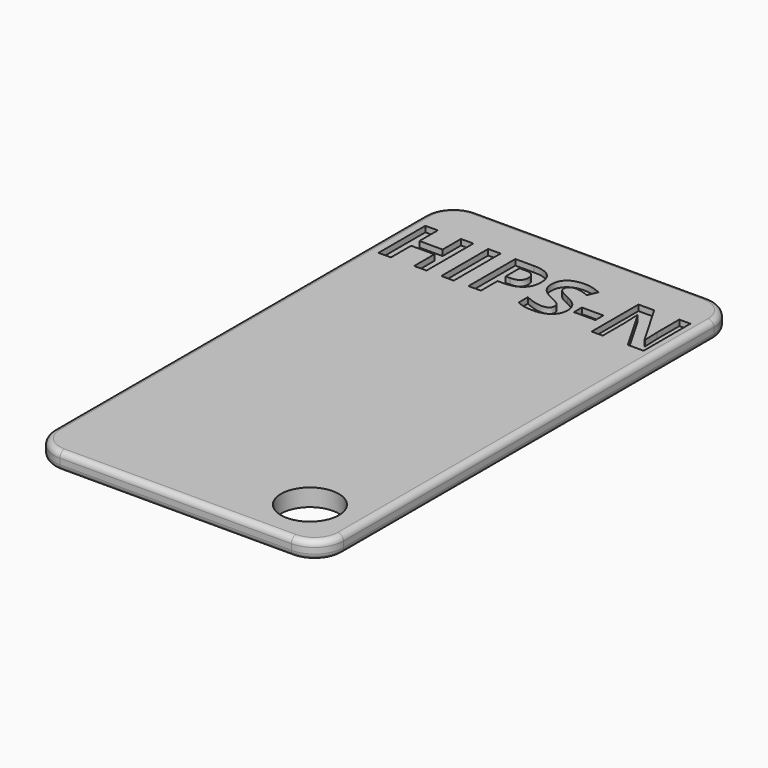
from build123d import *

# Parameters (mm, degrees)
F0_W         = 90
F0_H         = 50
F1_DEPTH     = 3
F2_R         = 1
F3_T1_DEPTH  = 3
F3_T4_ANGLE  = 90
F3_T6_ANGLE  = 90
F3_T8_ANGLE  = 90
F3_T10_ANGLE = 90
F3_T12_ANGLE = 90
F3_T14_ANGLE = 90
F3_T16_ANGLE = 90
F3_T18_ANGLE = 90
F5_ANGLE     = 90
F6_TEXT_SIZE = 14.1815160188
F7_DEPTH     = 1
F8_R         = 5
F9_DEPTH     = 3


# Not quite as in the source:
# - a fillet or chamfer that OpenCascade refuses, or shapes differently, is made with other operations: its cross-section is extruded or revolved along the edge and cut away or added
# - Text() gives the source's letters only with a copy of the font that has no kerning and outlines rounded to 1/6400 em; it was checked with that copy


with BuildPart() as f1:
    # F0 (on Top) → F1 (new body)
    with BuildSketch(Plane.XY):
        Rectangle(F0_W, F0_H)
    extrude(amount=F1_DEPTH)

    # F2
    f2_edges = [f1.edges().sort_by_distance(p)[0] for p in [
        (0, 25, 3),
        (-45, 0, 3),
        (0, -25, 3),
        (45, 0, 3),
        (0, 25, 0),
        (-45, 0, 0),
        (0, -25, 0),
        (45, 0, 0),
    ]]
    fillet(f2_edges, radius=F2_R)

    # F3: fillet of radius 5 on 4 edges, made by hand

    # F3_s2 → F3_t1 (cut)
    with BuildSketch(Plane.XY):
        with BuildLine():
            ThreePointArc((45, -20), (43.5355339059, -23.5355339059), (40, -25))
            Line((40, -25), (45, -25))
            Line((45, -25), (45, -20))
        make_face()
        with BuildLine():
            ThreePointArc((40, 25), (43.5355339059, 23.5355339059), (45, 20))
            Line((45, 20), (45, 25))
            Line((45, 25), (40, 25))
        make_face()
        with BuildLine():
            ThreePointArc((-40, 25), (-43.5355339059, 23.5355339059), (-45, 20))
            Line((-45, 20), (-45, 25))
            Line((-45, 25), (-40, 25))
        make_face()
        with BuildLine():
            ThreePointArc((-45, -20), (-43.5355339059, -23.5355339059), (-40, -25))
            Line((-40, -25), (-45, -25))
            Line((-45, -25), (-45, -20))
        make_face()
    extrude(amount=F3_T1_DEPTH, mode=Mode.SUBTRACT)

    # F3_s3 → F3_t4 (revolve, cut)
    with BuildSketch(Plane.YZ.offset(-40)):
        with BuildLine():
            ThreePointArc((-24, 0), (-24.7071067812, 0.2928932188), (-25, 1))
            Line((-25, 1), (-25, 0))
            Line((-25, 0), (-24, 0))
        make_face()
    revolve(axis=Axis((-40, -20, 0), (0, 0, -1)), revolution_arc=F3_T4_ANGLE, mode=Mode.SUBTRACT)

    # F3_s5 → F3_t6 (revolve, cut)
    with BuildSketch(Plane.XZ.offset(20)):
        with BuildLine():
            ThreePointArc((-44, 3), (-44.7071067812, 2.7071067812), (-45, 2))
            Line((-45, 2), (-45, 3))
            Line((-45, 3), (-44, 3))
        make_face()
    revolve(axis=Axis((-40, -20, 3), (0, 0, 1)), revolution_arc=F3_T6_ANGLE, mode=Mode.SUBTRACT)

    # F3_s7 → F3_t8 (revolve, cut)
    with BuildSketch(Plane.XZ.offset(-20)):
        with BuildLine():
            ThreePointArc((-44, 0), (-44.7071067812, 0.2928932188), (-45, 1))
            Line((-45, 1), (-45, 0))
            Line((-45, 0), (-44, 0))
        make_face()
    revolve(axis=Axis((-40, 20, 0), (0, 0, -1)), revolution_arc=F3_T8_ANGLE, mode=Mode.SUBTRACT)

    # F3_s9 → F3_t10 (revolve, cut)
    with BuildSketch(Plane.YZ.offset(-40)):
        with BuildLine():
            ThreePointArc((24, 3), (24.7071067812, 2.7071067812), (25, 2))
            Line((25, 2), (25, 3))
            Line((25, 3), (24, 3))
        make_face()
    revolve(axis=Axis((-40, 20, 3), (0, 0, 1)), revolution_arc=F3_T10_ANGLE, mode=Mode.SUBTRACT)

    # F3_s11 → F3_t12 (revolve, cut)
    with BuildSketch(Plane.YZ.offset(40)):
        with BuildLine():
            ThreePointArc((24, 0), (24.7071067812, 0.2928932188), (25, 1))
            Line((25, 1), (25, 0))
            Line((25, 0), (24, 0))
        make_face()
    revolve(axis=Axis((40, 20, 0), (0, 0, -1)), revolution_arc=F3_T12_ANGLE, mode=Mode.SUBTRACT)

    # F3_s13 → F3_t14 (revolve, cut)
    with BuildSketch(Plane.XZ.offset(-20)):
        with BuildLine():
            ThreePointArc((44, 3), (44.7071067812, 2.7071067812), (45, 2))
            Line((45, 2), (45, 3))
            Line((45, 3), (44, 3))
        make_face()
    revolve(axis=Axis((40, 20, 3), (0, 0, 1)), revolution_arc=F3_T14_ANGLE, mode=Mode.SUBTRACT)

    # F3_s15 → F3_t16 (revolve, cut)
    with BuildSketch(Plane.XZ.offset(20)):
        with BuildLine():
            ThreePointArc((44, 0), (44.7071067812, 0.2928932188), (45, 1))
            Line((45, 1), (45, 0))
            Line((45, 0), (44, 0))
        make_face()
    revolve(axis=Axis((40, -20, 0), (0, 0, -1)), revolution_arc=F3_T16_ANGLE, mode=Mode.SUBTRACT)

    # F3_s17 → F3_t18 (revolve, cut)
    with BuildSketch(Plane.YZ.offset(40)):
        with BuildLine():
            ThreePointArc((-24, 3), (-24.7071067812, 2.7071067812), (-25, 2))
            Line((-25, 2), (-25, 3))
            Line((-25, 3), (-24, 3))
        make_face()
    revolve(axis=Axis((40, -20, 3), (0, 0, 1)), revolution_arc=F3_T18_ANGLE, mode=Mode.SUBTRACT)


with BuildPart() as f1_1:
    # F5: moved
    add(f1.part.rotate(Axis((0, 0, 16.4477843791), (0, 0, 1)), F5_ANGLE))

    # F6 (on face) → F7 (cut)
    with BuildSketch(Plane.XY.offset(3)):
        with Locations((-24, 27.2197566456)):
            Text('HIPS-N', F6_TEXT_SIZE, font='Open Sans', font_style=FontStyle.BOLD, text_align=(TextAlign.LEFT, TextAlign.BOTTOM))
    extrude(amount=-F7_DEPTH, mode=Mode.SUBTRACT)

    # F8 (on face) → F9 (cut)
    with BuildSketch(Plane.XY.offset(3)):
        with Locations((16, -36)):
            Circle(F8_R)
    extrude(amount=-F9_DEPTH, mode=Mode.SUBTRACT)


solid = f1_1.part
